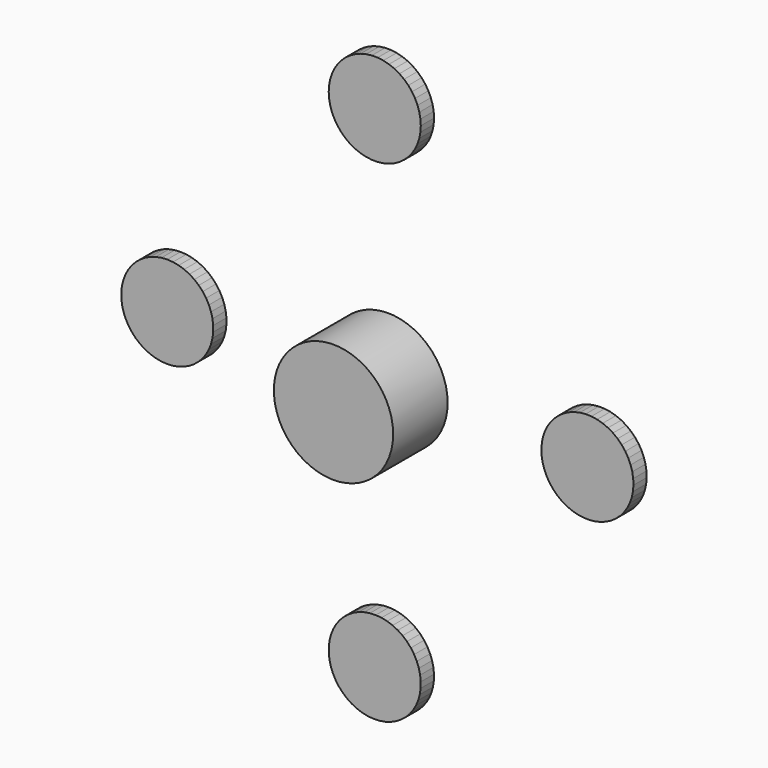
from build123d import *

# Parameters (mm, degrees)
F0_R     = 16.45568758
F1_DEPTH = 18.796
F7_DEPTH = 4.572
F8_T     = -2.54
F8_2_T   = -2.54
F8_3_T   = -2.54
F8_4_T   = -2.54


# Not quite as in the source:
# - the program builds the solid bodies; features that only make, move or delete a surface that nothing else refers to are left out


with BuildPart() as f1:
    # F0 (on Front) → F1 (new body)
    with BuildSketch(Plane.XZ):
        Circle(F0_R)
    extrude(amount=F1_DEPTH)


with BuildPart() as f7:
    # F6 (on Front) → F7 (new body)
    with BuildSketch(Plane.XZ):
        Polygon((-7.242148221, -57.2248721426), (-8.4926061045, -58.2148189753), (-9.6091305165, -59.3536837115), (-10.5741132, -60.623505774), (-11.3723358017, -62.0042593104), (-11.9912098743, -63.4741690124), (-12.420975404, -65.0100535262), (-12.6548547316, -66.5876910353), (-12.6891594405, -68.1822012538), (-12.5233485248, -69.768437803), (-12.1600369219, -71.3213847851), (-11.6049542726, -72.8165512984), (-10.866854562, -74.2303576738), (-9.9573780634, -75.5405073402), (-8.8908677644, -76.7263384548), (-7.6841431697, -77.7691497525), (-6.356235047, -78.6524954761), (-4.9280853005, -79.3624447359), (-3.4222167049, -79.8878012081), (-1.8623777075, -80.2202797071), (-0.2731679012, -80.3546368485), (1.3203499261, -80.2887537398), (2.8930450464, -80.0236693971), (4.420115118, -79.5635643588), (5.8774773338, -78.9156947562), (7.242148221, -78.0902778799), (8.4926061045, -77.1003310472), (9.6091305165, -75.961466311), (10.5741132, -74.6916442485), (11.3723358017, -73.3108907121), (11.9912098743, -71.8409810101), (12.420975404, -70.3050964963), (12.6548547316, -68.7274589873), (12.6891594405, -67.1329487687), (12.5233485248, -65.5467122195), (12.1600369219, -63.9937652374), (11.6049542726, -62.4985987241), (10.866854562, -61.0847923487), (9.9573780634, -59.7746426823), (8.8908677644, -58.5888115677), (7.6841431697, -57.5460002701), (6.356235047, -56.6626545464), (4.9280853005, -55.9527052866), (3.4222167049, -55.4273488145), (1.8623777075, -55.0948703154), (0.2731679012, -54.9605131741), (-1.3203499261, -55.0263962827), (-2.8930450464, -55.2914806254), (-4.420115118, -55.7515856637), (-5.8774773338, -56.3994552663), align=None)
    extrude(amount=F7_DEPTH)

    # F8#3
    f8_3_openings = [f7.faces().sort_by_distance(p)[0] for p in [
        (0, 0, -67.657575),
    ]]
    offset(amount=F8_3_T, openings=f8_3_openings)


with BuildPart() as f7b:
    # F6 (on Front) → F7, piece 2 (new body)
    with BuildSketch(Plane.XZ):
        Polygon((47.6938120835, 6.3816573596), (46.9805603647, 4.9551540699), (46.4517211187, 3.4505050404), (46.1156344564, 1.8914394852), (45.9776006652, 0.3025447995), (46.0397966204, -1.2911211985), (46.3012414546, -2.8644254439), (46.7578120267, -4.392555989), (47.402307946, -5.8514133021), (48.2245651269, -7.2179903319), (49.2116160823, -8.4707353424), (50.3478944292, -9.5898917964), (51.6154803791, -10.557809928), (52.9943833444, -11.3592250902), (54.4628572017, -11.981498487), (55.9977432411, -12.4148164952), (57.5748353927, -12.6523454311), (59.1692619712, -12.6903393214), (60.755877917, -12.5281989797), (62.3096613489, -12.1684814562), (63.8061081739, -11.6168597109), (65.2216185318, -10.8820331485), (66.5338689785, -9.9755904227), (67.7221645405, -8.9118266768), (68.7677650872, -7.7075181006), (69.6541808731, -6.3816573596), (70.367432592, -4.9551540699), (70.8962718379, -3.4505050404), (71.2323585002, -1.8914394852), (71.3703922915, -0.3025447995), (71.3081963363, 1.2911211985), (71.046751502, 2.8644254439), (70.5901809299, 4.392555989), (69.9456850106, 5.8514133021), (69.1234278298, 7.2179903319), (68.1363768743, 8.4707353424), (67.0000985275, 9.5898917964), (65.7325125776, 10.557809928), (64.3536096122, 11.3592250902), (62.8851357549, 11.981498487), (61.3502497156, 12.4148164952), (59.773157564, 12.6523454311), (58.1787309855, 12.6903393214), (56.5921150396, 12.5281989797), (55.0383316077, 12.1684814562), (53.5418847827, 11.6168597109), (52.1263744249, 10.8820331485), (50.8141239782, 9.9755904227), (49.6258284161, 8.9118266768), (48.5802278694, 7.7075181006), align=None)
    extrude(amount=F7_DEPTH)

    # F8
    f8_openings = [f7b.faces().sort_by_distance(p)[0] for p in [
        (58.673996, 0, 0),
    ]]
    offset(amount=F8_T, openings=f8_openings)


with BuildPart() as f7c:
    # F6 (on Front) → F7, piece 3 (new body)
    with BuildSketch(Plane.XZ):
        Polygon((0.797439598, 80.6132597898), (-0.797439598, 80.6132597898), (-2.3797426952, 80.413368423), (-3.9245158286, 80.0167380957), (-5.4073970029, 79.429623905), (-6.8050002962, 78.6612849926), (-8.0952846698, 77.723838522), (-9.2579015683, 76.632068584), (-10.2745158286, 75.4031930428), (-11.1290948366, 74.0565919998), (-11.8081613708, 72.6135021578), (-12.3010061463, 71.0966819057), (-12.5998567067, 69.530052405), (-12.7, 67.9383203387), (-12.5998567067, 66.3465882725), (-12.3010061463, 64.7799587717), (-11.8081613708, 63.2631385196), (-11.1290948366, 61.8200486776), (-10.2745158286, 60.4734476346), (-9.2579015683, 59.2445720934), (-8.0952846698, 58.1528021555), (-6.8050002962, 57.2153556849), (-5.4073970029, 56.4470167724), (-3.9245158286, 55.8599025818), (-2.3797426952, 55.4632722545), (-0.797439598, 55.2633808877), (0.797439598, 55.2633808877), (2.3797426952, 55.4632722545), (3.9245158286, 55.8599025818), (5.4073970029, 56.4470167724), (6.8050002962, 57.2153556849), (8.0952846698, 58.1528021555), (9.2579015683, 59.2445720934), (10.2745158286, 60.4734476346), (11.1290948366, 61.8200486776), (11.8081613708, 63.2631385196), (12.3010061463, 64.7799587717), (12.5998567067, 66.3465882725), (12.7, 67.9383203387), (12.5998567067, 69.530052405), (12.3010061463, 71.0966819057), (11.8081613708, 72.6135021578), (11.1290948366, 74.0565919998), (10.2745158286, 75.4031930428), (9.2579015683, 76.632068584), (8.0952846698, 77.723838522), (6.8050002962, 78.6612849926), (5.4073970029, 79.429623905), (3.9245158286, 80.0167380957), (2.3797426952, 80.413368423), align=None)
    extrude(amount=F7_DEPTH)

    # F8#2
    f8_2_openings = [f7c.faces().sort_by_distance(p)[0] for p in [
        (0, 0, 67.93832),
    ]]
    offset(amount=F8_2_T, openings=f8_2_openings)


with BuildPart() as f7d:
    # F6 (on Front) → F7, piece 4 (new body)
    with BuildSketch(Plane.XZ):
        Polygon((-44.5744871089, -0.797439598), (-44.5744871089, 0.797439598), (-44.7743784756, 2.3797426952), (-45.1710088029, 3.9245158286), (-45.7581229936, 5.4073970029), (-46.526461906, 6.8050002962), (-47.4639083766, 8.0952846698), (-48.5556783146, 9.2579015683), (-49.7845538558, 10.2745158286), (-51.1311548988, 11.1290948366), (-52.5742447408, 11.8081613708), (-54.0910649929, 12.3010061463), (-55.6576944936, 12.5998567067), (-57.2494265599, 12.7), (-58.8411586262, 12.5998567067), (-60.4077881269, 12.3010061463), (-61.924608379, 11.8081613708), (-63.367698221, 11.1290948366), (-64.714299264, 10.2745158286), (-65.9431748052, 9.2579015683), (-67.0349447431, 8.0952846698), (-67.9723912138, 6.8050002962), (-68.7407301262, 5.4073970029), (-69.3278443168, 3.9245158286), (-69.7244746441, 2.3797426952), (-69.9243660109, 0.797439598), (-69.9243660109, -0.797439598), (-69.7244746441, -2.3797426952), (-69.3278443168, -3.9245158286), (-68.7407301262, -5.4073970029), (-67.9723912138, -6.8050002962), (-67.0349447431, -8.0952846698), (-65.9431748052, -9.2579015683), (-64.714299264, -10.2745158286), (-63.367698221, -11.1290948366), (-61.924608379, -11.8081613708), (-60.4077881269, -12.3010061463), (-58.8411586262, -12.5998567067), (-57.2494265599, -12.7), (-55.6576944936, -12.5998567067), (-54.0910649929, -12.3010061463), (-52.5742447408, -11.8081613708), (-51.1311548988, -11.1290948366), (-49.7845538558, -10.2745158286), (-48.5556783146, -9.2579015683), (-47.4639083766, -8.0952846698), (-46.526461906, -6.8050002962), (-45.7581229936, -5.4073970029), (-45.1710088029, -3.9245158286), (-44.7743784756, -2.3797426952), align=None)
    extrude(amount=F7_DEPTH)

    # F8#4
    f8_4_openings = [f7d.faces().sort_by_distance(p)[0] for p in [
        (-57.249427, 0, 0),
    ]]
    offset(amount=F8_4_T, openings=f8_4_openings)


solid = Compound([f1.part, f7.part, f7b.part, f7c.part, f7d.part])
